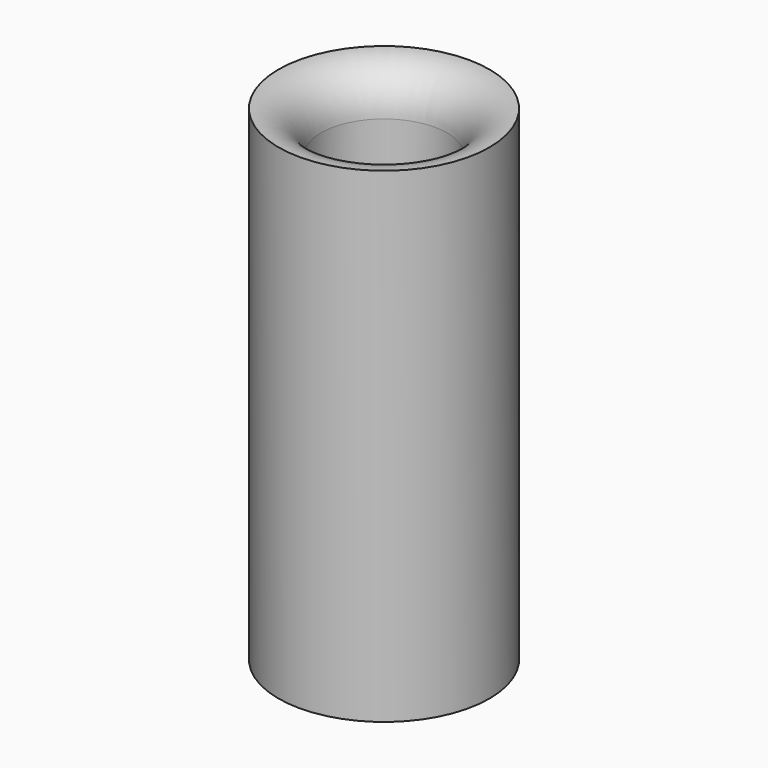
from build123d import *

# Parameters (mm, degrees)
F0_R      = 5
F0_R_2    = 3.81
F1_DEPTH  = 28
F3_R      = 4.2
F4_DEPTH  = 10
F5_R      = 6.6272432787
F6_DEPTH  = 10
F2_R      = 4.2
F7_DEPTH  = 17
F9_DEPTH  = 6
F10_R     = 4.2
F11_DEPTH = 2
F12_R     = 5
F12_R_2   = 3
F13_DEPTH = 5
F14_R     = 1.99999


# Not quite as in the source:
# - a fillet or chamfer is up to 0.001 mm smaller than in the source, because OpenCascade refuses the exact size


with BuildPart() as f1:
    # F0 (on Top) → F1 (new body)
    with BuildSketch(Plane.XY):
        Circle(F0_R)
        Circle(F0_R_2, mode=Mode.SUBTRACT)
    extrude(amount=F1_DEPTH)

    # F3 (on face) → F4 (cut)
    with BuildSketch(Plane(origin=(0, 0, 0), x_dir=(1, 0, 0), z_dir=(0, 0, -1))):
        with Locations((0.1565692156, 0)):
            Circle(F3_R)
    extrude(amount=-F4_DEPTH, mode=Mode.SUBTRACT)

    # F5 (on face) → F6 (cut)
    with BuildSketch(Plane(origin=(0, 0, 0), x_dir=(1, 0, 0), z_dir=(0, 0, -1))):
        with Locations((-0.2925955923, 0)):
            Circle(F5_R)
    extrude(amount=-F6_DEPTH, mode=Mode.SUBTRACT)

    # F2 (on face) → F7 (cut)
    with BuildSketch(Plane.XY.offset(28)):
        Circle(F2_R)
    extrude(amount=-F7_DEPTH, mode=Mode.SUBTRACT)

    # F8 (on face) → F9 (join)
    with BuildSketch(Plane.XY.offset(28)):
        with BuildLine():
            ThreePointArc((1.8834823008, 3.7539971261), (0.2542086961, 4.2354191199), (-1.4209507588, 3.9523282937))
            ThreePointArc((-1.4209507588, 3.9523282937), (0.1766375517, 2.9429916253), (1.8834823008, 3.7539971261))
        make_face()
    extrude(amount=-F9_DEPTH)

    # F10 (on face) → F11 (cut)
    with BuildSketch(Plane.XY.offset(28)):
        Circle(F10_R)
    extrude(amount=-F11_DEPTH, mode=Mode.SUBTRACT)

    # F12 (on face) → F13 (join)
    with BuildSketch(Plane.XY.offset(28)):
        Circle(F12_R)
        Circle(F12_R_2, mode=Mode.SUBTRACT)
    extrude(amount=F13_DEPTH)

    # F14 (radius 2 in the source; OpenCascade refuses exactly that, so slightly less here)
    f14_edges = [f1.edges().sort_by_distance(p)[0] for p in [
        (-3, 0, 33),
    ]]
    fillet(f14_edges, radius=F14_R)


solid = f1.part
